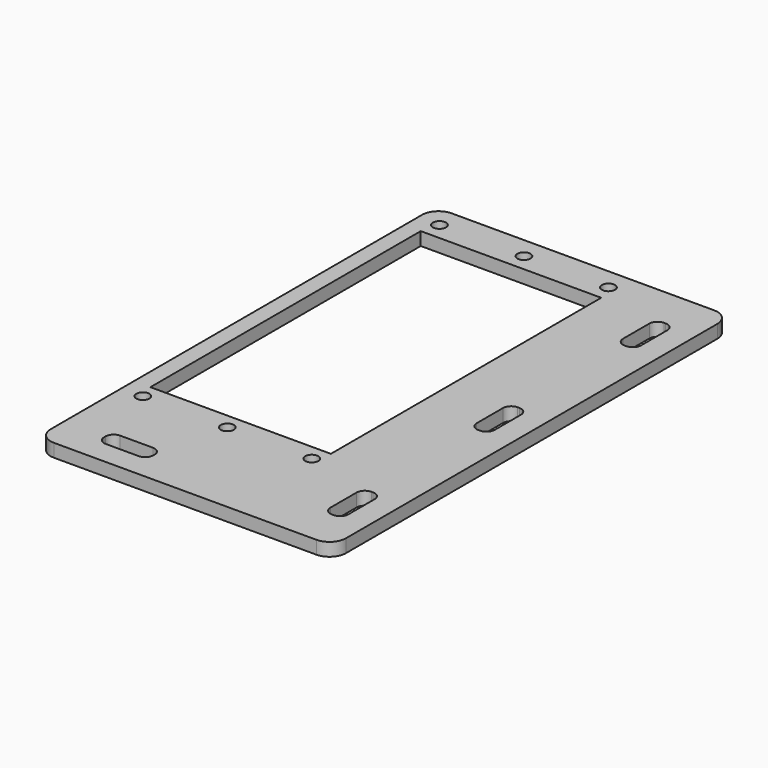
from build123d import *

# Parameters (mm, degrees)
F0_W     = 15
F0_H     = 5.5
F0_R     = 2
F0_W_2   = 5.5
F0_H_2   = 15
F0_W_3   = 55
F0_H_3   = 103
F1_DEPTH = 4
F2_R     = 2.5
F3_R     = 5


# Not quite as in the source:
# - a feature names something its author has since deleted; it is built from what else it names


with BuildPart() as f1:
    # F0 (on Top) → F1 (new body)
    with BuildSketch(Plane.XY):
        Polygon((57.5, 63.25), (32.5, 63.25), (-32.5, 63.25), (-32.5, -63.25), (-32.5, -88.25), (57.5, -88.25), align=None)
        with Locations((-12.5, -78.25)):
            Rectangle(F0_W, F0_H, mode=Mode.SUBTRACT)
        with Locations((-26, -56.25)):
            Circle(F0_R, mode=Mode.SUBTRACT)
        with Locations((-0.25, -56.25)):
            Circle(F0_R, mode=Mode.SUBTRACT)
        with Locations((25.5, -56.25)):
            Circle(F0_R, mode=Mode.SUBTRACT)
        with Locations((47.5, -68.25)):
            Rectangle(F0_W_2, F0_H_2, mode=Mode.SUBTRACT)
        Rectangle(F0_W_3, F0_H_3, mode=Mode.SUBTRACT)
        with Locations((-26, 56.75)):
            Circle(F0_R, mode=Mode.SUBTRACT)
        with Locations((-0.25, 56.75)):
            Circle(F0_R, mode=Mode.SUBTRACT)
        with Locations((47.5, -12.5)):
            Rectangle(F0_W_2, F0_H_2, mode=Mode.SUBTRACT)
        with Locations((25.5, 56.75)):
            Circle(F0_R, mode=Mode.SUBTRACT)
        with Locations((47.5, 43.25)):
            Rectangle(F0_W_2, F0_H_2, mode=Mode.SUBTRACT)
    extrude(amount=F1_DEPTH)

    # F2
    f2_edges = [f1.edges().sort_by_distance(p)[0] for p in [
        (-20, -81, 2),
        (-20, -75.5, 2),
        (-5, -75.5, 2),
        (-5, -81, 2),
        (50.25, -60.75, 2),
        (50.25, -75.75, 2),
        (44.75, -75.75, 2),
        (44.75, -60.75, 2),
        (44.75, -5, 2),
        (50.25, -5, 2),
        (50.25, -20, 2),
        (44.75, -20, 2),
        (44.75, 35.75, 2),
        (44.75, 50.75, 2),
        (50.25, 50.75, 2),
        (50.25, 35.75, 2),
    ]]
    fillet(f2_edges, radius=F2_R)

    # F3
    f3_edges = [f1.edges().sort_by_distance(p)[0] for p in [
        (-32.5, 63.25, 2),
        (-32.5, -88.25, 2),
        (57.5, -88.25, 2),
        (57.5, 63.25, 2),
    ]]
    fillet(f3_edges, radius=F3_R)


solid = f1.part
